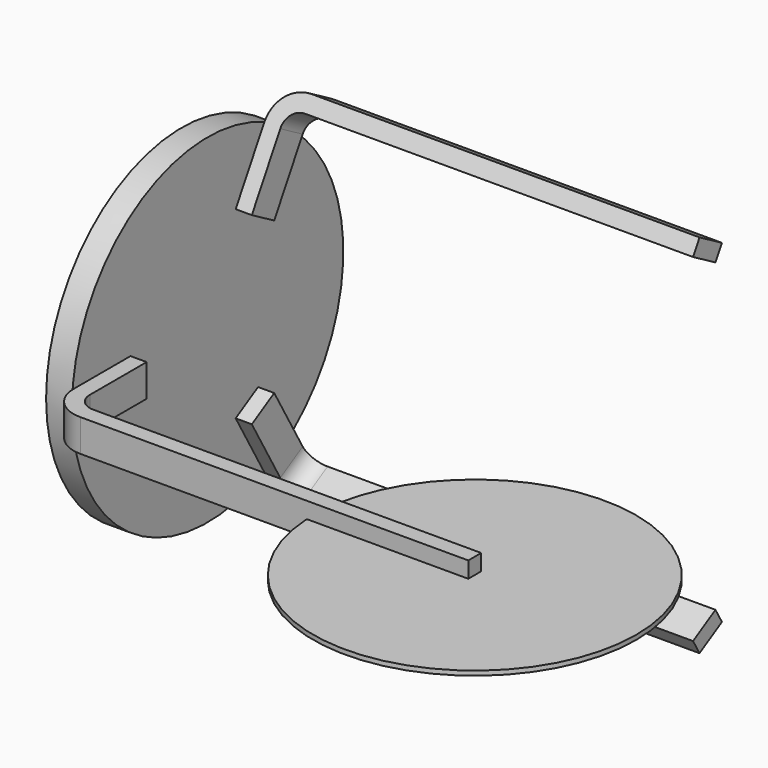
from build123d import *

# Parameters (mm, degrees)
F0_R      = 6350
F1_DEPTH  = 177.8
F6_W      = 635
F6_H      = 1270
F10_COUNT = 3
F12_R     = 6663.9545311895
F13_DEPTH = 1016


with BuildPart() as f1:
    # F0 (on Top) → F1 (new body)
    with BuildSketch(Plane.XY):
        Circle(F0_R)
    extrude(amount=-F1_DEPTH)


with BuildPart() as f7:
    # F7: sweep along a path in F5
    with BuildLine(Plane.XY) as f7_path:
        Line((0, 0), (-15240, 0))
        ThreePointArc((-15240, 0), (-15958.4204896855, 297.5795103145), (-16256, 1016))
        Line((-16256, 1016), (-16256, 3810))
    # F6 (on face) → F7 (sweep)
    with BuildSketch(Plane.YZ):
        Rectangle(F6_W, F6_H)
    sweep(path=f7_path.line)


with BuildPart() as f10_1:
    # F10: instance of F7
    add(f7.part.rotate(Axis((-7049.0123681202, 7620, 0), (1, 0, 0)), 1 * 360 / F10_COUNT))


with BuildPart() as f10_2:
    # F10: instance of F7
    add(f7.part.rotate(Axis((-7049.0123681202, 7620, 0), (1, 0, 0)), 2 * 360 / F10_COUNT))


with BuildPart() as f7_1:
    add(f7.part)

    add(f10_1.part)  # F13 merges F10_1

    add(f10_2.part)  # F13 merges F10_2
    # F12 (on face) → F13 (join)
    with BuildSketch(Plane(origin=(-16573.5, 0, 0), x_dir=(0, -1, 0), z_dir=(-1, 0, 0))):
        with Locations((-7598.3817338374, 5.233656471)):
            Circle(F12_R)
    extrude(amount=F13_DEPTH)


solid = Compound([f1.part, f7_1.part])
